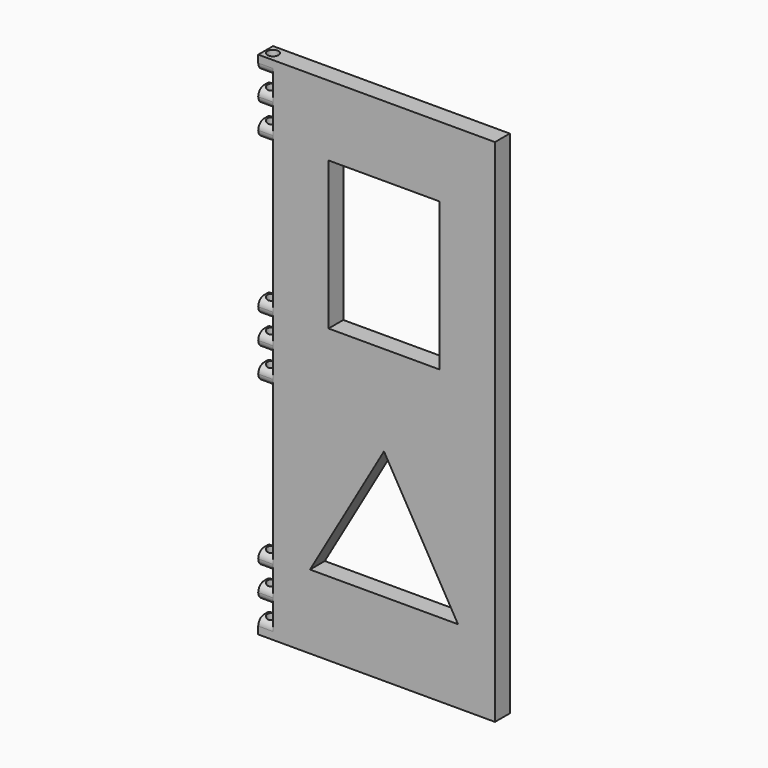
from build123d import *

# Parameters (mm, degrees)
F0_W        = 0.2
F0_H        = 0.2
F1_DEPTH    = 0.25
F3_DEPTH    = 25
F4_T1_DEPTH = 0.45


# Not quite as in the source:
# - a fillet or chamfer that OpenCascade refuses, or shapes differently, is made with other operations: its cross-section is extruded or revolved along the edge and cut away or added


with BuildPart() as f1:
    # F0 (on Front) → F1 (new body)
    with BuildSketch(Plane.XZ):
        Polygon((-1.5, -3.45), (1.5, -3.45), (1.5, 3.45), (-1.5, 3.45), (-1.5, 3.25), (-1.5, 3.05), (-1.5, 2.85), (-1.5, 2.65), (-1.5, 2.45), (-1.5, 0.55), (-1.5, 0.35), (-1.5, 0.15), (-1.5, -0.05), (-1.5, -0.25), (-1.5, -0.45), (-1.5, -2.45), (-1.5, -2.65), (-1.5, -2.85), (-1.5, -3.05), (-1.5, -3.25), align=None)
        Polygon((1, -2.45), (-1, -2.45), (0, -0.7179491924), align=None, mode=Mode.SUBTRACT)
        Polygon((-0.75, 0.5), (-0.75, 2.5), (0.75, 2.5), (0.75, 0.5), (0, 0.5), align=None, mode=Mode.SUBTRACT)
        with Locations((-1.6, -3.35)):
            Rectangle(F0_W, F0_H)
        with Locations((-1.6, -2.95)):
            Rectangle(F0_W, F0_H)
        with Locations((-1.6, -2.55)):
            Rectangle(F0_W, F0_H)
        with Locations((-1.6, -0.35)):
            Rectangle(F0_W, F0_H)
        with Locations((-1.6, 0.05)):
            Rectangle(F0_W, F0_H)
        with Locations((-1.6, 0.45)):
            Rectangle(F0_W, F0_H)
        with Locations((-1.6, 2.55)):
            Rectangle(F0_W, F0_H)
        with Locations((-1.6, 2.95)):
            Rectangle(F0_W, F0_H)
        with Locations((-1.6, 3.35)):
            Rectangle(F0_W, F0_H)
    extrude(amount=F1_DEPTH)

    # F2 (on face) → F3 (cut)
    with BuildSketch(Plane(origin=(0, 0, -3.45), x_dir=(1, 0, 0), z_dir=(0, 0, -1))):
        with BuildLine():
            ThreePointArc((-1.675, 0.125), (-1.6, 0.05), (-1.525, 0.125))
            ThreePointArc((-1.525, 0.125), (-1.6, 0.2), (-1.675, 0.125))
        make_face()
    extrude(amount=-F3_DEPTH, mode=Mode.SUBTRACT)

    # F4: fillet of radius 0.1 on 32 edges, made by hand

    # F4_s2 → F4_t1 (cut)
    with BuildSketch(Plane.YZ.offset(-1.95)):
        with BuildLine():
            ThreePointArc((-0.25, -2.55), (-0.2207106781, -2.4792893219), (-0.15, -2.45))
            Line((-0.15, -2.45), (-0.25, -2.45))
            Line((-0.25, -2.45), (-0.25, -2.55))
        make_face()
        with BuildLine():
            ThreePointArc((0, -2.55), (-0.0292893219, -2.4792893219), (-0.1, -2.45))
            Line((-0.1, -2.45), (0, -2.45))
            Line((0, -2.45), (0, -2.55))
        make_face()
        with BuildLine():
            ThreePointArc((-0.25, -2.55), (-0.2207106781, -2.6207106781), (-0.15, -2.65))
            Line((-0.15, -2.65), (-0.25, -2.65))
            Line((-0.25, -2.65), (-0.25, -2.55))
        make_face()
        with BuildLine():
            ThreePointArc((0, -2.55), (-0.0292893219, -2.6207106781), (-0.1, -2.65))
            Line((-0.1, -2.65), (0, -2.65))
            Line((0, -2.65), (0, -2.55))
        make_face()
        with BuildLine():
            ThreePointArc((-0.25, -2.95), (-0.2207106781, -2.8792893219), (-0.15, -2.85))
            Line((-0.15, -2.85), (-0.25, -2.85))
            Line((-0.25, -2.85), (-0.25, -2.95))
        make_face()
        with BuildLine():
            ThreePointArc((-0.25, -2.95), (-0.2207106781, -3.0207106781), (-0.15, -3.05))
            Line((-0.15, -3.05), (-0.25, -3.05))
            Line((-0.25, -3.05), (-0.25, -2.95))
        make_face()
        with BuildLine():
            ThreePointArc((0, -2.95), (-0.0292893219, -3.0207106781), (-0.1, -3.05))
            Line((-0.1, -3.05), (0, -3.05))
            Line((0, -3.05), (0, -2.95))
        make_face()
        with BuildLine():
            ThreePointArc((0, -2.95), (-0.0292893219, -2.8792893219), (-0.1, -2.85))
            Line((-0.1, -2.85), (0, -2.85))
            Line((0, -2.85), (0, -2.95))
        make_face()
        with BuildLine():
            ThreePointArc((0, -3.35), (-0.0292893219, -3.2792893219), (-0.1, -3.25))
            Line((-0.1, -3.25), (0, -3.25))
            Line((0, -3.25), (0, -3.35))
        make_face()
        with BuildLine():
            ThreePointArc((-0.25, -3.35), (-0.2207106781, -3.2792893219), (-0.15, -3.25))
            Line((-0.15, -3.25), (-0.25, -3.25))
            Line((-0.25, -3.25), (-0.25, -3.35))
        make_face()
        with BuildLine():
            ThreePointArc((0, -0.35), (-0.0292893219, -0.2792893219), (-0.1, -0.25))
            Line((-0.1, -0.25), (0, -0.25))
            Line((0, -0.25), (0, -0.35))
        make_face()
        with BuildLine():
            ThreePointArc((0, -0.35), (-0.0292893219, -0.4207106781), (-0.1, -0.45))
            Line((-0.1, -0.45), (0, -0.45))
            Line((0, -0.45), (0, -0.35))
        make_face()
        with BuildLine():
            ThreePointArc((-0.25, -0.35), (-0.2207106781, -0.2792893219), (-0.15, -0.25))
            Line((-0.15, -0.25), (-0.25, -0.25))
            Line((-0.25, -0.25), (-0.25, -0.35))
        make_face()
        with BuildLine():
            ThreePointArc((-0.25, -0.35), (-0.2207106781, -0.4207106781), (-0.15, -0.45))
            Line((-0.15, -0.45), (-0.25, -0.45))
            Line((-0.25, -0.45), (-0.25, -0.35))
        make_face()
        with BuildLine():
            ThreePointArc((-0.25, 0.05), (-0.2207106781, 0.1207106781), (-0.15, 0.15))
            Line((-0.15, 0.15), (-0.25, 0.15))
            Line((-0.25, 0.15), (-0.25, 0.05))
        make_face()
        with BuildLine():
            ThreePointArc((-0.25, 0.05), (-0.2207106781, -0.0207106781), (-0.15, -0.05))
            Line((-0.15, -0.05), (-0.25, -0.05))
            Line((-0.25, -0.05), (-0.25, 0.05))
        make_face()
        with BuildLine():
            ThreePointArc((0, 0.05), (-0.0292893219, 0.1207106781), (-0.1, 0.15))
            Line((-0.1, 0.15), (0, 0.15))
            Line((0, 0.15), (0, 0.05))
        make_face()
        with BuildLine():
            ThreePointArc((0, 0.05), (-0.0292893219, -0.0207106781), (-0.1, -0.05))
            Line((-0.1, -0.05), (0, -0.05))
            Line((0, -0.05), (0, 0.05))
        make_face()
        with BuildLine():
            ThreePointArc((0, 0.45), (-0.0292893219, 0.3792893219), (-0.1, 0.35))
            Line((-0.1, 0.35), (0, 0.35))
            Line((0, 0.35), (0, 0.45))
        make_face()
        with BuildLine():
            ThreePointArc((0, 0.45), (-0.0292893219, 0.5207106781), (-0.1, 0.55))
            Line((-0.1, 0.55), (0, 0.55))
            Line((0, 0.55), (0, 0.45))
        make_face()
        with BuildLine():
            ThreePointArc((-0.25, 0.45), (-0.2207106781, 0.3792893219), (-0.15, 0.35))
            Line((-0.15, 0.35), (-0.25, 0.35))
            Line((-0.25, 0.35), (-0.25, 0.45))
        make_face()
        with BuildLine():
            ThreePointArc((-0.25, 0.45), (-0.2207106781, 0.5207106781), (-0.15, 0.55))
            Line((-0.15, 0.55), (-0.25, 0.55))
            Line((-0.25, 0.55), (-0.25, 0.45))
        make_face()
        with BuildLine():
            ThreePointArc((-0.25, 2.55), (-0.2207106781, 2.6207106781), (-0.15, 2.65))
            Line((-0.15, 2.65), (-0.25, 2.65))
            Line((-0.25, 2.65), (-0.25, 2.55))
        make_face()
        with BuildLine():
            ThreePointArc((0, 2.55), (-0.0292893219, 2.6207106781), (-0.1, 2.65))
            Line((-0.1, 2.65), (0, 2.65))
            Line((0, 2.65), (0, 2.55))
        make_face()
        with BuildLine():
            ThreePointArc((-0.25, 2.95), (-0.2207106781, 3.0207106781), (-0.15, 3.05))
            Line((-0.15, 3.05), (-0.25, 3.05))
            Line((-0.25, 3.05), (-0.25, 2.95))
        make_face()
        with BuildLine():
            ThreePointArc((0, 2.95), (-0.0292893219, 3.0207106781), (-0.1, 3.05))
            Line((-0.1, 3.05), (0, 3.05))
            Line((0, 3.05), (0, 2.95))
        make_face()
        with BuildLine():
            ThreePointArc((-0.25, 2.95), (-0.2207106781, 2.8792893219), (-0.15, 2.85))
            Line((-0.15, 2.85), (-0.25, 2.85))
            Line((-0.25, 2.85), (-0.25, 2.95))
        make_face()
        with BuildLine():
            ThreePointArc((-0.25, 2.55), (-0.2207106781, 2.4792893219), (-0.15, 2.45))
            Line((-0.15, 2.45), (-0.25, 2.45))
            Line((-0.25, 2.45), (-0.25, 2.55))
        make_face()
        with BuildLine():
            ThreePointArc((-0.25, 3.35), (-0.2207106781, 3.2792893219), (-0.15, 3.25))
            Line((-0.15, 3.25), (-0.25, 3.25))
            Line((-0.25, 3.25), (-0.25, 3.35))
        make_face()
        with BuildLine():
            ThreePointArc((0, 3.35), (-0.0292893219, 3.2792893219), (-0.1, 3.25))
            Line((-0.1, 3.25), (0, 3.25))
            Line((0, 3.25), (0, 3.35))
        make_face()
        with BuildLine():
            ThreePointArc((0, 2.95), (-0.0292893219, 2.8792893219), (-0.1, 2.85))
            Line((-0.1, 2.85), (0, 2.85))
            Line((0, 2.85), (0, 2.95))
        make_face()
        with BuildLine():
            ThreePointArc((0, 2.55), (-0.0292893219, 2.4792893219), (-0.1, 2.45))
            Line((-0.1, 2.45), (0, 2.45))
            Line((0, 2.45), (0, 2.55))
        make_face()
    extrude(amount=F4_T1_DEPTH, mode=Mode.SUBTRACT)


solid = f1.part
